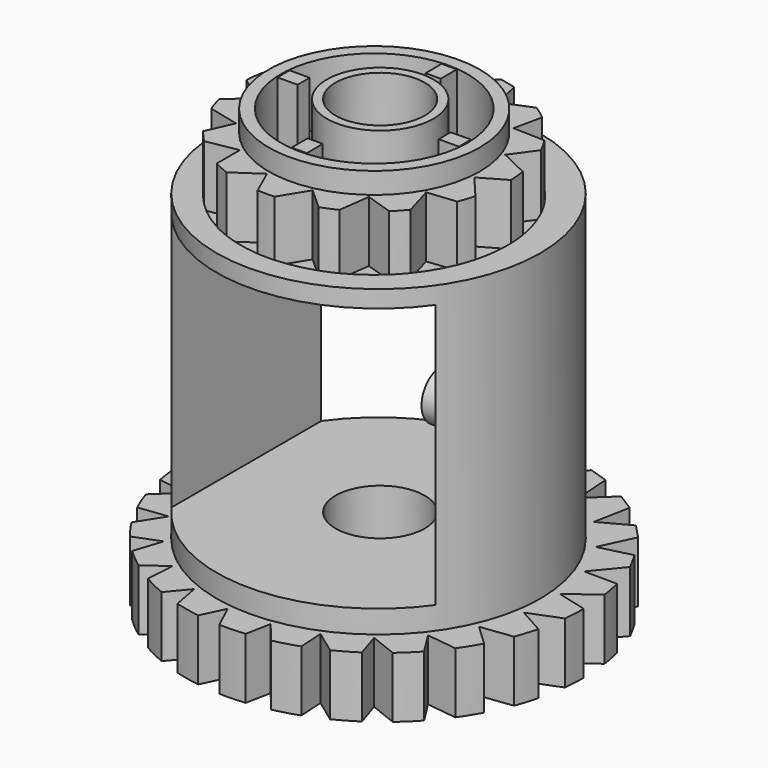
from build123d import *

# Parameters (mm, degrees)
F0_R      = 16.356674067
F1_DEPTH  = 5
F2_R      = 13.307352318
F3_DEPTH  = 25
F4_R      = 10.9792335934
F5_DEPTH  = 29.5873
F6_W      = 21.718283276
F6_H      = 21.718283276
F7_DEPTH  = 25
F8_DEPTH  = 25.34069
F9_R      = 3.6679757052
F10_DEPTH = 40.28341
F11_DEPTH = 25
F13_R     = 3.8770832675
F12_R     = 8.6799128885
F12_R_2   = 3.6679757052
F14_DEPTH = 1.73833
F15_R     = 7.6673406217
F16_DEPTH = 5
F17_R     = 4.3819915071
F18_DEPTH = 5.43034
F19_DEPTH = 40.71575
F21_DEPTH = 5
F22_R     = 8.6695894171
F23_DEPTH = 1.74844
F24_R     = 7.7631402001
F25_DEPTH = 5
F26_R     = 4.1288697506
F27_DEPTH = 5.35521
F28_DEPTH = 25
F29_R     = 13.5636947973
F29_R_2   = 8.6695894171
F30_DEPTH = 3
F32_DEPTH = 5
F33_R     = 2.0359532686
F34_DEPTH = 5
F35_W     = 0.7028965629
F35_H     = 2.1164277568
F35_W_2   = 2.1164277568
F35_H_2   = 0.7028965629
F36_DEPTH = 5
F38_DEPTH = 3
F40_DEPTH = 5


# Not quite as in the source:
# - ends of sketch curves that miss each other by under 0.0002 mm in the source are joined


with BuildPart() as f1:
    # F0 (on Top) → F1 (new body)
    with BuildSketch(Plane.XY):
        with Locations((0, -2.1748070139)):
            Circle(F0_R)
    extrude(amount=-F1_DEPTH)

    # F2 (on Top) → F3 (join)
    with BuildSketch(Plane.XY):
        with Locations((0, -2.8165236581)):
            Circle(F2_R)
    extrude(amount=F3_DEPTH)

    # F4 (on Top) → F5 (join)
    with BuildSketch(Plane.XY):
        with Locations((0, -3.2558445819)):
            Circle(F4_R)
    extrude(amount=F5_DEPTH)

    # F6 (on Front) → F7 (cut)
    with BuildSketch(Plane.XZ):
        with Locations((0, 12.7306869254)):
            Rectangle(F6_W, F6_H)
    extrude(amount=-F7_DEPTH, mode=Mode.SUBTRACT)

    # F6 (on Front) → F8 (cut)
    with BuildSketch(Plane.XZ):
        with Locations((0, 12.7306869254)):
            Rectangle(F6_W, F6_H)
    extrude(amount=F8_DEPTH, mode=Mode.SUBTRACT)

    # F9 (on Top) → F10 (cut)
    with BuildSketch(Plane.XY):
        with Locations((0, -2.6447952259)):
            Circle(F9_R)
    extrude(amount=F10_DEPTH, mode=Mode.SUBTRACT)

    # F9 (on Top) → F11 (cut)
    with BuildSketch(Plane.XY):
        with Locations((0, -2.6447952259)):
            Circle(F9_R)
    extrude(amount=-F11_DEPTH, mode=Mode.SUBTRACT)

    # F13 (on face) + F12 (on face) → F14 (join)
    with BuildSketch(Plane.XY.offset(29.5873)):
        with Locations((0, -2.7154064737)):
            Circle(F13_R)
    with BuildSketch(Plane.XY.offset(29.5873)):
        with Locations((0, -3.2558445819)):
            Circle(F12_R)
        with Locations((0, -2.6447952259)):
            Circle(F12_R_2, mode=Mode.SUBTRACT)
    extrude(amount=F14_DEPTH)

    # F15 (on face) → F16 (cut)
    with BuildSketch(Plane.XY.offset(31.32563)):
        with Locations((0, -3.2558445819)):
            Circle(F15_R)
    extrude(amount=-F16_DEPTH, mode=Mode.SUBTRACT)

    # F17 (on face) → F18 (join)
    with BuildSketch(Plane.XY.offset(26.32563)):
        with Locations((0, -2.6447952259)):
            Circle(F17_R)
    extrude(amount=F18_DEPTH)

    # F9 (on Top) → F19 (cut)
    with BuildSketch(Plane.XY):
        with Locations((0, -2.6447952259)):
            Circle(F9_R)
    extrude(amount=F19_DEPTH, mode=Mode.SUBTRACT)

    # F20 (on face) → F21 (cut)
    with BuildSketch(Plane.XY.offset(29.5873)):
        with BuildLine():
            Line((-10.8024524707, -1.2935523212), (-8.5437586025, -0.5596581957))
            Line((-8.5437586025, -0.5596581957), (-9.7790416548, 1.7355394558))
            ThreePointArc((-9.7790416548, 1.7355394558), (-10.4016020092, 0.2584470879), (-10.8024524707, -1.2935523212))
        make_face()
        with BuildLine():
            ThreePointArc((-10.9637778716, -2.6734829421), (-10.9317274643, -4.276092074), (-10.6666675528, -5.8569546555))
            Line((-10.6666675528, -5.8569546555), (-8.9017496624, -4.2678154491))
            Line((-8.9017496624, -4.2678154491), (-10.9637778716, -2.6734829421))
        make_face()
        with BuildLine():
            Line((-8.6865189115, -9.9706014277), (-7.7205473357, -7.800993746))
            Line((-7.7205473357, -7.800993746), (-10.2527772917, -7.1832009581))
            ThreePointArc((-10.2527772917, -7.1832009581), (-9.5716579291, -8.6342211758), (-8.6865189115, -9.9706014277))
        make_face()
        with BuildLine():
            Line((-1.7883504378, -12.0346278005), (-3.9418525172, -13.5030573263))
            ThreePointArc((-3.9418525172, -13.5030573263), (-2.4077765387, -13.9678090346), (-0.822378862, -14.2042354821))
            Line((-0.822378862, -14.2042354821), (-1.7883504378, -12.0346278005))
        make_face()
        with BuildLine():
            Line((-5.2043922357, -12.9232057396), (-5.2043922357, -10.5482744611))
            Line((-5.2043922357, -10.5482744611), (-7.7689783744, -11.0138433777))
            ThreePointArc((-7.7689783744, -11.0138433777), (-6.5565617822, -12.0623801035), (-5.2043922357, -12.9232057396))
        make_face()
        with BuildLine():
            Line((1.9369133975, -12.0030497686), (0.5668554507, -14.2204350984))
            ThreePointArc((0.5668554507, -14.2204350984), (2.1573351423, -14.0210419968), (3.701831288, -13.592188975))
            Line((3.701831288, -13.592188975), (1.9369133975, -12.0030497686))
        make_face()
        with BuildLine():
            Line((7.5859611782, -11.1928946195), (5.32726731, -10.459000494))
            Line((5.32726731, -10.459000494), (4.9775489616, -13.04193556))
            ThreePointArc((4.9775489616, -13.04193556), (6.3494239785, -12.2128745271), (7.5859611782, -11.1928946195))
        make_face()
        with BuildLine():
            Line((10.1584094645, -7.4212122067), (7.796488308, -7.6694601236))
            Line((7.796488308, -7.6694601236), (8.5275790373, -10.1713319877))
            ThreePointArc((8.5275790373, -10.1713319877), (9.443639726, -8.8559552078), (10.1584094645, -7.4212122067))
        make_face()
        with BuildLine():
            Line((10.974376468, -2.9292998904), (8.9176256486, -4.1167655297))
            Line((8.9176256486, -4.1167655297), (10.6031132269, -6.1049778176))
            ThreePointArc((10.6031132269, -6.1049778176), (10.8847973622, -4.6927707043), (10.9792335934, -3.2558445819))
            ThreePointArc((10.9792335934, -3.2558445819), (10.9780192449, -3.0925541755), (10.974376468, -2.9292998904))
        make_face()
        with BuildLine():
            Line((9.8927740812, 1.5061498822), (8.4968245005, -0.4152098826))
            Line((8.4968245005, -0.4152098826), (10.8452728133, -1.5459826275))
            ThreePointArc((10.8452728133, -1.5459826275), (10.4807216099, 0.0149419954), (9.8927740812, 1.5061498822))
        make_face()
        with BuildLine():
            Line((7.1006211827, 5.1182075506), (6.606845205, 2.7951742186))
            Line((6.606845205, 2.7951742186), (9.2121862041, 2.717361897))
            ThreePointArc((9.2121862041, 2.717361897), (8.2442668669, 3.9950611633), (7.1006211827, 5.1182075506))
        make_face()
        with BuildLine():
            Line((3.0807063746, 7.2823155294), (3.5744823523, 4.9592821974))
            Line((3.5744823523, 4.9592821974), (5.9862289101, 5.9478847565))
            ThreePointArc((5.9862289101, 5.9478847565), (4.5823034858, 6.7214328555), (3.0807063746, 7.2823155294))
        make_face()
        with BuildLine():
            Line((-1.471890553, 7.6242798888), (-0.0759409723, 5.702920124))
            Line((-0.0759409723, 5.702920124), (1.7251982543, 7.5869992001))
            ThreePointArc((1.7251982543, 7.5869992001), (0.1280182031, 7.722642638), (-1.471890553, 7.6242798888))
        make_face()
        with BuildLine():
            Line((-5.7699842323, 6.0849718844), (-3.7132334129, 4.8975062452))
            Line((-3.7132334129, 4.8975062452), (-2.8341348525, 7.3512874497))
            ThreePointArc((-2.8341348525, 7.3512874497), (-4.3484025899, 6.8255722438), (-5.7699842323, 6.0849718844))
        make_face()
        with BuildLine():
            Line((-9.0703952192, 2.9305518543), (-6.7084740627, 2.6823039374))
            Line((-6.7084740627, 2.6823039374), (-6.9034202961, 5.2815062083))
            ThreePointArc((-6.9034202961, 5.2815062083), (-8.0729450712, 4.1853332937), (-9.0703952192, 2.9305518543))
        make_face()
    extrude(amount=-F21_DEPTH, mode=Mode.SUBTRACT)

    # F22 (on face) → F23 (join)
    with BuildSketch(Plane(origin=(0, 0, -5), x_dir=(1, 0, 0), z_dir=(0, 0, -1))):
        with Locations((0, 2.6447952259)):
            Circle(F22_R)
    extrude(amount=F23_DEPTH)

    # F24 (on face) → F25 (cut)
    with BuildSketch(Plane(origin=(0, 0, -6.74844), x_dir=(1, 0, 0), z_dir=(0, 0, -1))):
        with Locations((0, 2.6447952259)):
            Circle(F24_R)
    extrude(amount=-F25_DEPTH, mode=Mode.SUBTRACT)

    # F26 (on face) → F27 (join)
    with BuildSketch(Plane(origin=(0, 0, -1.74844), x_dir=(1, 0, 0), z_dir=(0, 0, -1))):
        with Locations((0, 2.6447952259)):
            Circle(F26_R)
    extrude(amount=F27_DEPTH)

    # F9 (on Top) → F28 (cut)
    with BuildSketch(Plane.XY):
        with Locations((0, -2.6447952259)):
            Circle(F9_R)
    extrude(amount=-F28_DEPTH, mode=Mode.SUBTRACT)

    # F29 (on face) → F30 (cut)
    with BuildSketch(Plane(origin=(0, 0, -5), x_dir=(1, 0, 0), z_dir=(0, 0, -1))):
        with Locations((0, 2.6447952259)):
            Circle(F29_R)
        with Locations((0, 2.6447952259)):
            Circle(F29_R_2, mode=Mode.SUBTRACT)
    extrude(amount=-F30_DEPTH, mode=Mode.SUBTRACT)

    # F31 (on face) → F32 (cut)
    with BuildSketch(Plane(origin=(0, 0, -5), x_dir=(1, 0, 0), z_dir=(0, 0, -1))):
        with BuildLine():
            Line((-16.3178522764, 1.0485372338), (-13.8794748915, 2.0271305025))
            Line((-13.8794748915, 2.0271305025), (-16.3133042358, 3.3651395072))
            ThreePointArc((-16.3133042358, 3.3651395072), (-16.3566425453, 2.2069189894), (-16.3178522764, 1.0485372338))
        make_face()
        with BuildLine():
            Line((-15.5060753604, -3.0311908203), (-13.2898186948, -1.4051494691))
            Line((-13.2898186948, -1.4051494691), (-16.1052116938, -0.6822794096))
            ThreePointArc((-16.1052116938, -0.6822794096), (-15.8492180725, -1.867849665), (-15.5060753604, -3.0311908203))
        make_face()
        with BuildLine():
            Line((-11.865114313, -4.5829565208), (-14.8954160245, -4.5829565208))
            ThreePointArc((-14.8954160245, -4.5829565208), (0.1463029011, -14.181212734), (15.0139179322, -4.315420629))
            Line((15.0139179322, -4.315420629), (14.257366836, -5.6848315114))
            Line((14.257366836, -5.6848315114), (11.5917852755, -5.0136541668))
            Line((11.5917852755, -5.0136541668), (12.8820249914, -7.7555531324))
            Line((12.8820249914, -7.7555531324), (11.737951506, -8.9688039201))
            Line((11.737951506, -8.9688039201), (9.3230291099, -7.6558096684))
            Line((9.3230291099, -7.6558096684), (9.8908510282, -10.6324364054))
            Line((9.8908510282, -10.6324364054), (8.4809975136, -11.5230511825))
            Line((8.4809975136, -11.5230511825), (6.4684727377, -9.6507402815))
            Line((6.4684727377, -9.6507402815), (6.2781985189, -12.6750623847))
            Line((6.2781985189, -12.6750623847), (4.6911512566, -13.1870805495))
            Line((4.6911512566, -13.1870805495), (3.207478434, -10.8730971789))
            Line((3.207478434, -10.8730971789), (2.2710637071, -13.7550853679))
            Line((2.2710637071, -13.7550853679), (0.6065427132, -13.8563349359))
            Line((0.6065427132, -13.8563349359), (-0.255053536, -11.2460751812))
            Line((-0.255053536, -11.2460751812), (-1.8787703899, -13.8046435388))
            Line((-1.8787703899, -13.8046435388), (-3.5161771395, -13.4887626273))
            Line((-3.5161771395, -13.4887626273), (-3.7015595544, -10.7462387087))
            Line((-3.7015595544, -10.7462387087), (-5.9105544336, -12.8206229754))
            Line((-5.9105544336, -12.8206229754), (-7.4179626509, -12.1074595437))
            Line((-7.4179626509, -12.1074595437), (-6.9154829725, -9.4049943254))
            Line((-6.9154829725, -9.4049943254), (-9.5709566048, -10.8648533085))
            Line((-9.5709566048, -10.8648533085), (-10.8536502877, -9.799218038))
            Line((-10.8536502877, -9.799218038), (-9.6948811621, -7.3066173485))
            Line((-9.6948811621, -7.3066173485), (-12.6299803729, -8.0602227392))
            Line((-12.6299803729, -8.0602227392), (-13.6073631599, -6.709073413))
            Line((-13.6073631599, -6.709073413), (-11.865114313, -4.5829565208))
        make_face()
        with BuildLine():
            Line((13.1321869406, -1.890290124), (15.0563959385, -4.2162592412))
            ThreePointArc((15.0563959385, -4.2162592412), (15.495738277, -3.0618791313), (15.8467182651, -1.8776375273))
            Line((15.8467182651, -1.8776375273), (13.1321869406, -1.890290124))
        make_face()
        with BuildLine():
            Line((13.8474450034, 1.5180300102), (16.1861180082, -0.1811153869))
            ThreePointArc((16.1861180082, -0.1811153869), (16.3139793307, 0.9937630131), (16.356674067, 2.1748070139))
            Line((16.356674067, 2.1748070139), (13.8474450034, 1.5180300102))
        make_face()
        with BuildLine():
            Line((13.6926171693, 4.9971489468), (16.2565295333, 3.9820242298))
            ThreePointArc((16.2565295333, 3.9820242298), (16.0934851344, 5.0972242944), (15.8540306122, 6.1985490385))
            Line((15.8540306122, 6.1985490385), (13.6926171693, 4.9971489468))
        make_face()
        with BuildLine():
            Line((12.6774318405, 8.3284608479), (15.2845798343, 7.9991014623))
            ThreePointArc((15.2845798343, 7.9991014623), (14.8692281634, 8.9899988937), (14.3897182052, 9.951489887))
            Line((14.3897182052, 9.951489887), (12.6774318405, 8.3284608479))
        make_face()
        with BuildLine():
            Line((10.8656768449, 11.3026471348), (13.3559435233, 11.6172409764))
            ThreePointArc((13.3559435233, 11.6172409764), (12.7368957073, 12.4369838919), (12.067612728, 13.2162520996))
            Line((12.067612728, 13.2162520996), (10.8656768449, 11.3026471348))
        make_face()
        with BuildLine():
            ThreePointArc((-15.5288889705, 7.3123544711), (-15.8403931596, 6.2519053796), (-16.079570356, 5.1728403194))
            Line((-16.079570356, 5.1728403194), (-13.5970326356, 5.4982206203))
            Line((-13.5970326356, 5.4982206203), (-15.5288889705, 7.3123544711))
        make_face()
        with BuildLine():
            Line((-14.8285768132, 9.0780016533), (-12.4602388128, 8.7900195263))
            Line((-12.4602388128, 8.7900195263), (-13.8172550128, 10.9283348995))
            ThreePointArc((-13.8172550128, 10.9283348995), (-14.3527646651, 10.0194824694), (-14.8285768132, 9.0780016533))
        make_face()
        with BuildLine():
            Line((-12.6651144954, 12.5254428085), (-10.5405223598, 11.6956913891))
            Line((-10.5405223598, 11.6956913891), (-11.2919496083, 14.008346661))
            ThreePointArc((-11.2919496083, 14.008346661), (-12.0014574563, 13.2881235962), (-12.6651144954, 12.5254428085))
        make_face()
        with BuildLine():
            Line((-9.7406673518, 15.3148293151), (-7.9585061217, 14.032662159))
            Line((-7.9585061217, 14.032662159), (-8.1062800049, 16.3814607725))
            ThreePointArc((-8.1062800049, 16.3814607725), (-8.9393964089, 15.8725432641), (-9.7406673518, 15.3148293151))
        make_face()
        with BuildLine():
            Line((-6.2447345217, 17.2924813485), (-4.8764276746, 15.6540913679))
            Line((-4.8764276746, 15.6540913679), (-4.4449577639, 17.9159358493))
            ThreePointArc((-4.4449577639, 17.9159358493), (-5.3539288535, 17.6304283979), (-6.2447345217, 17.2924813485))
        make_face()
        with BuildLine():
            Line((-2.3917046375, 18.3556764424), (-1.4879453424, 16.4580986553))
            Line((-1.4879453424, 16.4580986553), (-0.5161182944, 18.5233362579))
            ThreePointArc((-0.5161182944, 18.5233362579), (-1.4563262012, 18.4665196473), (-2.3917046375, 18.3556764424))
        make_face()
        with BuildLine():
            Line((1.5911550307, 18.4539044153), (1.9940300679, 16.3941652865))
            Line((1.9940300679, 16.3941652865), (3.4565756371, 18.1620791827))
            ThreePointArc((3.4565756371, 18.1620791827), (2.5280796497, 18.3349307702), (1.5911550307, 18.4539044153))
        make_face()
        with BuildLine():
            Line((5.4742854052, 17.5882098126), (5.3507132355, 15.4663084301))
            Line((5.3507132355, 15.4663084301), (7.2424008887, 16.8406999599))
            ThreePointArc((7.2424008887, 16.8406999599), (6.3693186699, 17.2404157376), (5.4742854052, 17.5882098126))
        make_face()
        with BuildLine():
            Line((9.0352581246, 15.8095016257), (8.3711914119, 13.7328287449))
            Line((8.3711914119, 13.7328287449), (10.6133747056, 14.6205719117))
            ThreePointArc((10.6133747056, 14.6205719117), (9.8422853794, 15.2388877333), (9.0352581246, 15.8095016257))
        make_face()
    extrude(amount=-F32_DEPTH, mode=Mode.SUBTRACT)

    # F33 (on face) → F34 (join)
    with BuildSketch(Plane(origin=(10.859141638, 0, 0), x_dir=(0, -1, 0), z_dir=(-1, 0, 0))):
        with Locations((3.6809588782, 12.7306869254)):
            Circle(F33_R)
    extrude(amount=F34_DEPTH)

    # F35 (on face) → F36 (join)
    with BuildSketch(Plane(origin=(0, 0, -1.74844), x_dir=(1, 0, 0), z_dir=(0, 0, -1))):
        with Locations((-0.3514482814, 9.2307459563)):
            Rectangle(F35_W, F35_H)
        with Locations((-6.5859507304, 2.2933469445)):
            Rectangle(F35_W_2, F35_H_2)
        with Locations((0.3514482814, -3.9411555044)):
            Rectangle(F35_W, F35_H)
        with Locations((6.5859507304, 2.9962435074)):
            Rectangle(F35_W_2, F35_H_2)
    extrude(amount=F36_DEPTH)

    # F37 (on face) → F38 (join)
    with BuildSketch(Plane(origin=(0, 0, -2), x_dir=(1, 0, 0), z_dir=(0, 0, -1))):
        Polygon((8.6739708204, 1.5510494122), (13.2924423087, 1.5510494122), (13.2441765163, 4.1028099367), (8.6739708204, 4.1028099367), align=None)
        Polygon((-1.0937458137, -10.6476470828), (1.4580147108, -10.5993812904), (1.4580147108, -6.0291755944), (-1.0937458137, -6.0291755944), align=None)
        Polygon((-8.6739708204, 3.7385410396), (-13.2924423087, 3.7385410396), (-13.2441765163, 1.1867805151), (-8.6739708204, 1.1867805151), align=None)
        Polygon((1.0937458137, 11.3187660463), (1.0937458137, 15.9372375347), (-1.4580147108, 15.8889717422), (-1.4580147108, 11.3187660463), align=None)
    extrude(amount=F38_DEPTH)

    # F39 (on face) → F40 (join)
    with BuildSketch(Plane.XY.offset(26.32563)):
        Polygon((5.8985368814, -2.7696313045), (5.8985368814, -4.0014818078), (7.5527862646, -4.0014818078), (7.5527862646, -2.7445326559), align=None)
        Polygon((0.4862132773, -9.1543814633), (-0.7456372259, -9.1543814633), (-0.7456372259, -10.8086308464), (0.5113119259, -10.8086308464), align=None)
        Polygon((0.7456372259, 4.2969416827), (-0.5113119259, 4.2969416827), (-0.4862132773, 2.6426922996), (0.7456372259, 2.6426922996), align=None)
        Polygon((-5.8985368814, -3.7420578592), (-5.8985368814, -2.510207356), (-7.5527862646, -2.510207356), (-7.5527862646, -3.7671565078), align=None)
    extrude(amount=F40_DEPTH)


solid = f1.part
